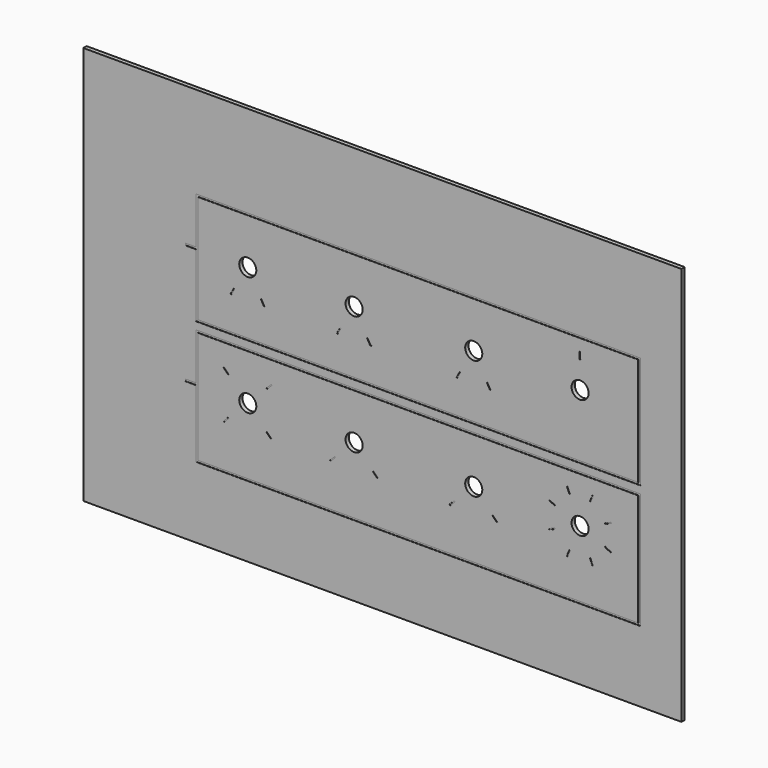
from build123d import *

# Parameters (mm, degrees)
F0_W     = 228.6
F0_H     = 152.4
F1_DEPTH = 1.5748
F3_D     = 6.5278
F5_W     = 0.381
F5_H     = 2.54
F6_DEPTH = 0.127
F7_W     = 168.275
F7_H     = 41.275
F7_W_2   = 3.96875
F7_H_2   = 0.79375
F7_H_3   = 42.8625
F8_DEPTH = 0.127


with BuildPart() as f1:
    # F0 (on Front) → F1 (new body)
    with BuildSketch(Plane.XZ):
        Rectangle(F0_W, F0_H)
    extrude(amount=F1_DEPTH)

    # F3 (through all)
    with Locations(Plane.XZ.offset(1.5748)):
        with Locations((-51.435, 22.86), (-10.795, 22.86), (34.925, 22.86), (75.565, 22.86), (75.565, -22.86), (34.925, -22.86), (-10.795, -22.86), (-51.435, -22.86)):
            Hole(F3_D / 2)

    # F5 (on face) → F6 (cut)
    with BuildSketch(Plane.XZ.offset(1.5748)):
        Polygon((-42.2090303616, -31.8165619547), (-44.0050815859, -30.0205107305), (-44.2744892695, -30.2899184141), (-42.4784380453, -32.0859696384), align=None)
        Polygon((-42.2090303616, -13.9034380453), (-42.4784380453, -13.6340303616), (-44.2744892695, -15.4300815859), (-44.0050815859, -15.6994892695), align=None)
        Polygon((80.3091585435, -10.9087876125), (79.3371426253, -13.2554416251), (79.6891407272, -13.4012440128), (80.6611566454, -11.0545900003), align=None)
        Polygon((85.0237559872, -18.7358592728), (85.1695583749, -19.0878573747), (87.5162123875, -18.1158414565), (87.3704099997, -17.7638433546), align=None)
        Polygon((85.1695583749, -26.6321426253), (85.0237559872, -26.9841407272), (87.3704099997, -27.9561566454), (87.5162123875, -27.6041585435), align=None)
        Polygon((79.6891407272, -32.3187559872), (79.3371426253, -32.4645583749), (80.3091585435, -34.8112123875), (80.6611566454, -34.6654099997), align=None)
        Polygon((71.7928573747, -32.4645583749), (71.4408592728, -32.3187559872), (70.4688433546, -34.6654099997), (70.8208414565, -34.8112123875), align=None)
        Polygon((66.1062440128, -26.9841407272), (65.9604416251, -26.6321426253), (63.6137876125, -27.6041585435), (63.7595900003, -27.9561566454), align=None)
        Polygon((65.9604416251, -19.0878573747), (66.1062440128, -18.7358592728), (63.7595900003, -17.7638433546), (63.6137876125, -18.1158414565), align=None)
        Polygon((71.4408592728, -13.4012440128), (71.7928573747, -13.2554416251), (70.8208414565, -10.9087876125), (70.4688433546, -11.0545900003), align=None)
        Polygon((27.4950815859, -30.0205107305), (25.6990303616, -31.8165619547), (25.9684380453, -32.0859696384), (27.7644892695, -30.2899184141), align=None)
        Polygon((44.1509696384, -31.8165619547), (42.3549184141, -30.0205107305), (42.0855107305, -30.2899184141), (43.8815619547, -32.0859696384), align=None)
        Polygon((-18.2249184141, -30.0205107305), (-20.0209696384, -31.8165619547), (-19.7515619547, -32.0859696384), (-17.9555107305, -30.2899184141), align=None)
        Polygon((-1.5690303616, -31.8165619547), (-3.3650815859, -30.0205107305), (-3.6344892695, -30.2899184141), (-1.8384380453, -32.0859696384), align=None)
        Polygon((-58.8649184141, -30.0205107305), (-60.6609696384, -31.8165619547), (-60.3915619547, -32.0859696384), (-58.5955107305, -30.2899184141), align=None)
        Polygon((-16.1184735337, 14.0204733668), (-17.3884735337, 11.8207688412), (-17.0585178549, 11.6302688412), (-15.7885178549, 13.8299733668), align=None)
        Polygon((-4.2015264663, 11.8207688412), (-5.4715264663, 14.0204733668), (-5.8014821451, 13.8299733668), (-4.5314821451, 11.6302688412), align=None)
        Polygon((-56.7584735337, 14.0204733668), (-58.0284735337, 11.8207688412), (-57.6985178549, 11.6302688412), (-56.4285178549, 13.8299733668), align=None)
        Polygon((-44.8415264663, 11.8207688412), (-46.1115264663, 14.0204733668), (-46.4414821451, 13.8299733668), (-45.1714821451, 11.6302688412), align=None)
        with Locations((75.565, 34.4469913886)):
            Rectangle(F5_W, F5_H)
        Polygon((40.2484735337, 14.0204733668), (40.0834956943, 13.9252233668), (41.3534956943, 11.7255188412), (41.5184735337, 11.8207688412), align=None)
        Polygon((41.3534956943, 11.7255188412), (40.0834956943, 13.9252233668), (39.9185178549, 13.8299733668), (41.1885178549, 11.6302688412), align=None)
        Polygon((29.6015264663, 14.0204733668), (28.3315264663, 11.8207688412), (28.6614821451, 11.6302688412), (29.9314821451, 13.8299733668), align=None)
        Polygon((-58.5955107305, -15.4300815859), (-60.3915619547, -13.6340303616), (-60.6609696384, -13.9034380453), (-58.8649184141, -15.6994892695), align=None)
    extrude(amount=-F6_DEPTH, mode=Mode.SUBTRACT)

    # F7 (on face) → F8 (cut)
    with BuildSketch(Plane.XZ.offset(1.5748)):
        Polygon((98.58375, 41.11625), (-71.27875, 41.11625), (-71.27875, 23.256875), (-71.27875, 22.463125), (-71.27875, -1.74625), (98.58375, -1.74625), align=None)
        with Locations((13.6525, 19.685)):
            Rectangle(F7_W, F7_H, mode=Mode.SUBTRACT)
        with Locations((-73.263125, 22.86)):
            Rectangle(F7_W_2, F7_H_2)
        Polygon((98.58375, -4.60375), (-71.27875, -4.60375), (-71.27875, -22.463125), (-71.27875, -23.256875), (-71.27875, -49.05375), (98.58375, -49.05375), align=None)
        with Locations((13.6525, -26.82875)):
            Rectangle(F7_W, F7_H_3, mode=Mode.SUBTRACT)
        with Locations((-73.263125, -22.86)):
            Rectangle(F7_W_2, F7_H_2)
    extrude(amount=-F8_DEPTH, mode=Mode.SUBTRACT)


solid = f1.part
